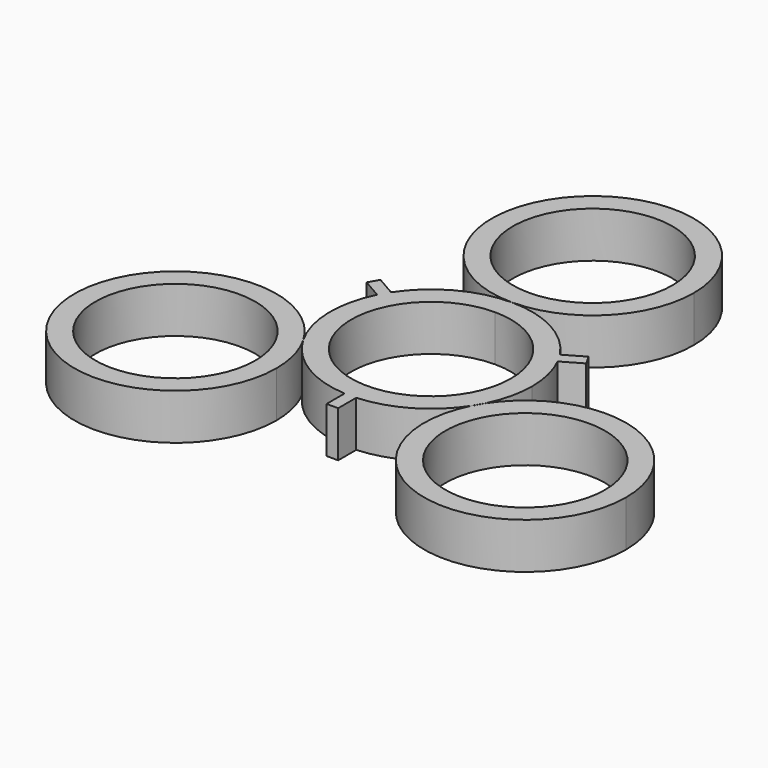
from build123d import *

# Parameters (mm, degrees)
F2_DEPTH = 6.35
F1_R     = 11.049
F6_W     = 1.6089215642
F6_H     = 3.1721480191
F7_DEPTH = 6.35


# Not quite as in the source:
# - the program builds the solid bodies; features that only make, move or delete a surface that nothing else refers to are left out


with BuildPart() as f2:
    # F1 (on face) → F2 (new body)
    with BuildSketch(Plane.XY):
        with BuildLine():
            ThreePointArc((0, 13.9879982162), (9.8782817332, 18.079716483), (13.97, 27.9579982162))
            ThreePointArc((13.97, 27.9579982162), (-9.8782817332, 37.8362799493), (0, 13.9879982162))
        make_face()
        with BuildLine():
            ThreePointArc((11.049, 27.94), (7.8128228253, 20.1271771747), (0, 16.891))
            ThreePointArc((0, 16.891), (-7.8128228253, 35.7528228253), (11.049, 27.94))
        make_face(mode=Mode.SUBTRACT)
    extrude(amount=F2_DEPTH)


with BuildPart() as f2b:
    # F1 (on face) → F2, piece 2 (new body)
    with BuildSketch(Plane.XY):
        with BuildLine():
            ThreePointArc((13.97, 0), (9.8782817332, 9.8782817332), (0, 13.97))
            ThreePointArc((0, 13.97), (-12.0758386026, 7.0238893815), (-12.1430715152, -6.9070047181))
            ThreePointArc((-12.1430715152, -6.9070047181), (-12.1001592972, -6.9808632821), (-12.0576994887, -7.0549828518))
            ThreePointArc((-12.0576994887, -7.0549828518), (-0.3379497641, -13.9659117123), (11.7023511261, -7.6299330352))
            ThreePointArc((11.7023511261, -7.6299330352), (12.063452241, -6.9631738679), (12.4601983994, -6.3169894607))
            ThreePointArc((12.4601983994, -6.3169894607), (13.5873078945, -3.2474550313), (13.97, 0))
        make_face()
        with BuildLine():
            ThreePointArc((11.049, 0), (-7.8128228253, -7.8128228253), (0, 11.049))
            ThreePointArc((0, 11.049), (7.8128228253, 7.8128228253), (11.049, 0))
        make_face(mode=Mode.SUBTRACT)
    extrude(amount=F2_DEPTH)

    # F6 (on Top) → F7 (join)
    with BuildSketch(Plane.XY):
        with Locations((0, -15.4868941754)):
            Rectangle(F6_W, F6_H)
        Polygon((14.3833937751, 9.2331675661), (11.636233006, 7.6470935566), (12.4406937881, 6.2537266093), (15.1878545572, 7.8398006188), align=None)
        Polygon((-15.1878545572, 7.8398006188), (-12.4406937881, 6.2537266093), (-11.636233006, 7.6470935566), (-14.3833937751, 9.2331675661), align=None)
    extrude(amount=F7_DEPTH)


with BuildPart() as f2c:
    # F1 (on face) → F2, piece 3 (new body)
    with BuildSketch(Plane.XY):
        with BuildLine():
            ThreePointArc((-12.0576994887, -7.0549828518), (-12.1006117068, -6.9811242878), (-12.1430715152, -6.9070047181))
            ThreePointArc((-12.1430715152, -6.9070047181), (-37.6842231186, -17.616767874), (-10.230771004, -13.9619875699))
            ThreePointArc((-10.230771004, -13.9619875699), (-10.6952238276, -10.3897200175), (-12.0576994887, -7.0549828518))
        make_face()
        with Locations((-24.1967497817, -13.97)):
            Circle(F1_R, mode=Mode.SUBTRACT)
    extrude(amount=F2_DEPTH)


with BuildPart() as f2d:
    # F1 (on face) → F2, piece 4 (new body)
    with BuildSketch(Plane.XY):
        with BuildLine():
            ThreePointArc((38.1325495255, -13.946922496), (28.1424398989, -0.5558294631), (12.4601983994, -6.3169894607))
            ThreePointArc((12.4601983994, -6.3169894607), (12.0990972845, -6.983748628), (11.7023511261, -7.6299330352))
            ThreePointArc((11.7023511261, -7.6299330352), (20.9150944942, -27.5342303905), (38.1325495255, -13.946922496))
        make_face()
        with Locations((24.1967497817, -13.97)):
            Circle(F1_R, mode=Mode.SUBTRACT)
    extrude(amount=F2_DEPTH)


solid = Compound([f2.part, f2b.part, f2c.part, f2d.part])
